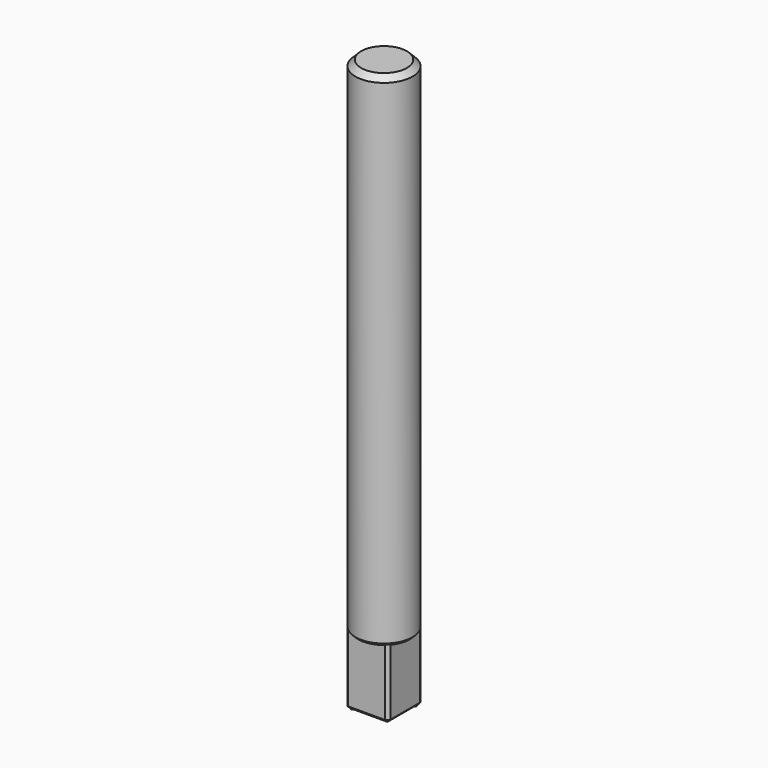
from build123d import *

# Parameters (mm, degrees)
F0_R         = 5
F1_DEPTH     = 100
F3_DEPTH     = 12
F4_SIZE      = 1
F5_SIZE      = 0.5
F6_T2_ANGLE  = 209.430321651
F6_T6_ANGLE  = 59.8137801049
F6_T12_ANGLE = 149.7566863334
F6_T18_ANGLE = 149.7566863334
F6_T25_ANGLE = 149.7566863334
F6_T31_ANGLE = 149.7566863334
F6_T38_ANGLE = 149.7566863334
F6_T45_ANGLE = 149.7566863334


# Not quite as in the source:
# - a fillet or chamfer that OpenCascade refuses, or shapes differently, is made with other operations: its cross-section is extruded or revolved along the edge and cut away or added


with BuildPart() as f1:
    # F0 (on Top) → F1 (new body)
    with BuildSketch(Plane.XY):
        Circle(F0_R)
    extrude(amount=F1_DEPTH)

    # F2 (on face) → F3 (cut)
    with BuildSketch(Plane(origin=(0, 0, 0), x_dir=(1, 0, 0), z_dir=(0, 0, -1))):
        with BuildLine():
            Line((-3.5, 3.5), (3.5, 3.5))
            Line((3.5, 3.5), (3.5, -3.5))
            Line((3.5, -3.5), (3.5307399131, -3.5403214072))
            ThreePointArc((3.5307399131, -3.5403214072), (4.6181002352, -1.9165464297), (5, 0))
            ThreePointArc((5, 0), (1.9130662834, 4.6195429855), (-3.5360709581, 3.5349967722))
            Line((-3.5360709581, 3.5349967722), (-3.5, 3.5))
        make_face()
    extrude(amount=-F3_DEPTH, mode=Mode.SUBTRACT)

    # F4
    f4_edges = [f1.edges().sort_by_distance(p)[0] for p in [
        (-5, 0, 100),
    ]]
    chamfer(f4_edges, length=F4_SIZE)

    # F5
    f5_edges = [f1.edges().sort_by_distance(p)[0] for p in [
        (0, -3.5, 0),
        (3.5, 0, 0),
        (3.5, -3.5, 6),
    ]]
    chamfer(f5_edges, length=F5_SIZE)

    # F6: chamfer of 0.5 on 3 edges, made by hand

    # F6_s1 → F6_t2 (revolve, cut)
    with BuildSketch(Plane(origin=(0, 0, 0), x_dir=(0, 0, 1), z_dir=(0.5048185175, -0.8632255003, 0))):
        Polygon((0.5, -5), (0, -4.5), (0, -5), align=None)
    revolve(axis=Axis((0, 0, 0), (0, 0, 1)), revolution_arc=F6_T2_ANGLE, mode=Mode.SUBTRACT)


with BuildPart() as f6_tool4:
    # F6_s5 → F6_t6 (revolve)
    with BuildSketch(Plane(origin=(0, 0, 0), x_dir=(0, 0, 1), z_dir=(-0.8643957574, 0.5028120669, 0))):
        Polygon((12, 4.5), (12.5, 5), (12, 5), align=None)
    revolve(axis=Axis((0, 0, 12), (0, 0, -1)), revolution_arc=F6_T6_ANGLE)

    split(bisect_by=Plane.YZ.offset(3.5), keep=Keep.TOP)

    split(bisect_by=Plane(origin=(0.5259878903, -0.4009984555, 0), x_dir=(0, 0, 1), z_dir=(0.7952525516, -0.6062783018, 0)), keep=Keep.TOP)


with BuildPart() as f1_1:
    add(f1.part)

    # F6_t3: cut F6_tool4
    add(f6_tool4.part, mode=Mode.SUBTRACT)


with BuildPart() as f6_tool10:
    # F6_s11 → F6_t12 (revolve)
    with BuildSketch(Plane.XZ):
        Polygon((4.5, 12), (5, 12.5), (5, 12), align=None)
    revolve(axis=Axis((0, 0, 12), (0, 0, -1)), revolution_arc=F6_T12_ANGLE)

    split(bisect_by=Plane(origin=(3.25, -3.25, 0), x_dir=(0, 0, 1), z_dir=(-0.7071067812, 0.7071067812, 0)), keep=Keep.TOP)

    split(bisect_by=Plane.YZ.offset(3.5), keep=Keep.TOP)


with BuildPart() as f1_2:
    add(f1_1.part)

    # F6_t9: cut F6_tool10
    add(f6_tool10.part, mode=Mode.SUBTRACT)


with BuildPart() as f6_tool16:
    # F6_s17 → F6_t18 (revolve)
    with BuildSketch(Plane.XZ):
        Polygon((4.5, 12), (5, 12.5), (5, 12), align=None)
    revolve(axis=Axis((0, 0, 12), (0, 0, -1)), revolution_arc=F6_T18_ANGLE)

    split(bisect_by=Plane.XZ.offset(3.5), keep=Keep.BOTTOM)

    split(bisect_by=Plane(origin=(3.25, -3.25, 0), x_dir=(0, 0, 1), z_dir=(0.7071067812, -0.7071067812, 0)), keep=Keep.TOP)

    split(bisect_by=Plane.YZ.offset(3.5), keep=Keep.TOP)


with BuildPart() as f1_3:
    add(f1_2.part)

    # F6_t15: cut F6_tool16
    add(f6_tool16.part, mode=Mode.SUBTRACT)


with BuildPart() as f6_tool23:
    # F6_s24 → F6_t25 (revolve)
    with BuildSketch(Plane.XZ):
        Polygon((4.5, 12), (5, 12.5), (5, 12), align=None)
    revolve(axis=Axis((0, 0, 12), (0, 0, -1)), revolution_arc=F6_T25_ANGLE)

    split(bisect_by=Plane.XZ.offset(3.5), keep=Keep.TOP)

    split(bisect_by=Plane.YZ.offset(3.5), keep=Keep.TOP)


with BuildPart() as f1_4:
    add(f1_3.part)

    # F6_t22: cut F6_tool23
    add(f6_tool23.part, mode=Mode.SUBTRACT)


with BuildPart() as f6_tool29:
    # F6_s30 → F6_t31 (revolve)
    with BuildSketch(Plane.XZ):
        Polygon((4.5, 12), (5, 12.5), (5, 12), align=None)
    revolve(axis=Axis((0, 0, 12), (0, 0, -1)), revolution_arc=F6_T31_ANGLE)

    split(bisect_by=Plane.XZ.offset(3.5), keep=Keep.BOTTOM)

    split(bisect_by=Plane(origin=(3.25, -3.25, 0), x_dir=(0, 0, 1), z_dir=(0.7071067812, -0.7071067812, 0)), keep=Keep.TOP)

    split(bisect_by=Plane.YZ.offset(3.5), keep=Keep.BOTTOM)


with BuildPart() as f1_5:
    add(f1_4.part)

    # F6_t28: cut F6_tool29
    add(f6_tool29.part, mode=Mode.SUBTRACT)


with BuildPart() as f6_tool36:
    # F6_s37 → F6_t38 (revolve)
    with BuildSketch(Plane.XZ):
        Polygon((4.5, 12), (5, 12.5), (5, 12), align=None)
    revolve(axis=Axis((0, 0, 12), (0, 0, -1)), revolution_arc=F6_T38_ANGLE)

    split(bisect_by=Plane.XZ.offset(3.5), keep=Keep.TOP)

    split(bisect_by=Plane(origin=(3.25, -3.25, 0), x_dir=(0, 0, 1), z_dir=(-0.7071067812, 0.7071067812, 0)), keep=Keep.TOP)

    split(bisect_by=Plane(origin=(0.0520908408, -0.0536897095, 0), x_dir=(0, 0, 1), z_dir=(0.6963393518, -0.7177126913, 0)), keep=Keep.TOP)


with BuildPart() as f1_6:
    add(f1_5.part)

    # F6_t35: cut F6_tool36
    add(f6_tool36.part, mode=Mode.SUBTRACT)


with BuildPart() as f6_tool43:
    # F6_s44 → F6_t45 (revolve)
    with BuildSketch(Plane.XZ):
        Polygon((4.5, 12), (5, 12.5), (5, 12), align=None)
    revolve(axis=Axis((0, 0, 12), (0, 0, -1)), revolution_arc=F6_T45_ANGLE)

    split(bisect_by=Plane.XZ.offset(3.5), keep=Keep.TOP)

    split(bisect_by=Plane(origin=(3.25, -3.25, 0), x_dir=(0, 0, 1), z_dir=(0.7071067812, -0.7071067812, 0)), keep=Keep.TOP)

    split(bisect_by=Plane.YZ.offset(3.5), keep=Keep.BOTTOM)


with BuildPart() as f1_7:
    add(f1_6.part)

    # F6_t42: cut F6_tool43
    add(f6_tool43.part, mode=Mode.SUBTRACT)


solid = f1_7.part
